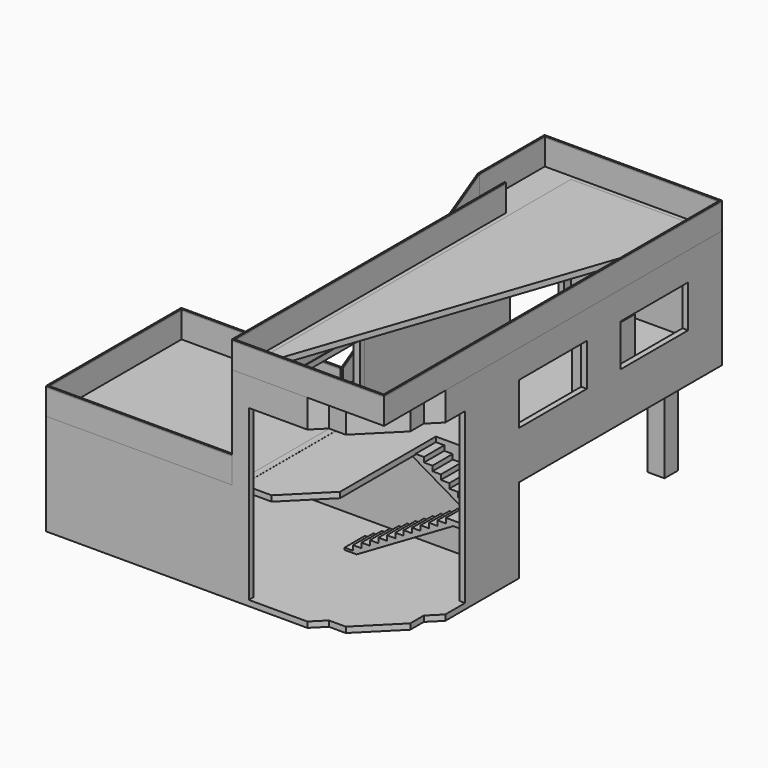
from build123d import *

# Parameters (mm, degrees)
F0_W      = 12192
F0_H      = 6096
F1_DEPTH  = 3657.6
F2_W      = 5486.4
F2_H      = 9144
F2_H_2    = 6096
F3_DEPTH  = 3657.6
F4_W      = 304.8
F4_H      = 101.6
F4_W_2    = 2997.2
F4_H_2    = 203.2
F5_DEPTH  = 914.4
F7_DEPTH  = 914.4
F8_DEPTH  = 50.8
F10_DEPTH = 914.4
F11_DEPTH = 50.8
F13_DEPTH = 50.8
F14_W     = 4876.8
F14_H     = 2438.4
F15_DEPTH = 228.6
F16_T     = -203.2
F17_W     = 3657.6
F17_H     = 6096
F18_DEPTH = 4876.8
F19_W     = 3048
F19_H     = 1524
F20_DEPTH = 203.2
F21_DEPTH = 609.6
F22_DEPTH = 203.2
F24_DEPTH = 203.2
F26_W     = 609.6
F26_H     = 609.6
F27_DEPTH = 3048
F28_W     = 2438.4
F28_H     = 3454.4
F29_DEPTH = 203.2
F30_DEPTH = 50.8
F31_W     = 228.6
F31_H     = 4876.8
F32_DEPTH = 2.54
F34_DEPTH = 7315.201
F36_DEPTH = 812.8
F38_DEPTH = 1828.8
F39_W     = 2090.0571428571
F39_H     = 914.4
F40_DEPTH = 1244.6
F41_W     = 4470.4
F41_H     = 914.4
F42_DEPTH = 2032
F44_DEPTH = 203.2
F46_DEPTH = 203.2
F49_DEPTH = 2438.4


with BuildPart() as f1:
    # F0 (on Top) → F1 (new body)
    with BuildSketch(Plane.XY):
        with Locations((-6096, 3048)):
            Rectangle(F0_W, F0_H)
    extrude(amount=F1_DEPTH)

    # F2 (on face) → F3 (join)
    with BuildSketch(Plane.XY.offset(3657.6)):
        with Locations((-2743.2, 10668)):
            Rectangle(F2_W, F2_H)
        with Locations((-2743.2, 3048)):
            Rectangle(F2_W, F2_H_2)
    extrude(amount=F3_DEPTH)

    # F4 (on face) → F5 (join)
    with BuildSketch(Plane(origin=(-5486.4, 0, 0), x_dir=(0, -1, 0), z_dir=(-1, 0, 0))):
        with Locations((-6248.4, 3784.6)):
            Rectangle(F4_W, F4_H)
        with Locations((-6553.2, 3962.4)):
            Rectangle(F4_W, F4_H)
        with Locations((-6858, 4140.2)):
            Rectangle(F4_W, F4_H)
        with Locations((-7162.8, 4318)):
            Rectangle(F4_W, F4_H)
        with Locations((-7467.6, 4495.8)):
            Rectangle(F4_W, F4_H)
        with Locations((-7772.4, 4673.6)):
            Rectangle(F4_W, F4_H)
        with Locations((-8077.2, 4851.4)):
            Rectangle(F4_W, F4_H)
        with Locations((-8382, 5029.2)):
            Rectangle(F4_W, F4_H)
        with Locations((-8686.8, 5207)):
            Rectangle(F4_W, F4_H)
        with Locations((-8991.6, 5384.8)):
            Rectangle(F4_W, F4_H)
        with Locations((-9296.4, 5562.6)):
            Rectangle(F4_W, F4_H)
        with Locations((-9601.2, 5740.4)):
            Rectangle(F4_W, F4_H)
        with Locations((-9906, 5918.2)):
            Rectangle(F4_W, F4_H)
        with Locations((-10210.8, 6096)):
            Rectangle(F4_W, F4_H)
        with Locations((-10515.6, 6273.8)):
            Rectangle(F4_W, F4_H)
        with Locations((-10820.4, 6451.6)):
            Rectangle(F4_W, F4_H)
        with Locations((-11125.2, 6629.4)):
            Rectangle(F4_W, F4_H)
        with Locations((-11430, 6807.2)):
            Rectangle(F4_W, F4_H)
        with Locations((-11734.8, 6985)):
            Rectangle(F4_W, F4_H)
        with Locations((-12039.6, 7162.8)):
            Rectangle(F4_W, F4_H)
        with Locations((-13741.4, 7213.6)):
            Rectangle(F4_W_2, F4_H_2)
    extrude(amount=F5_DEPTH)

    # F14 (on face) → F15 (cut)
    with BuildSketch(Plane(origin=(-5486.4, 0, 0), x_dir=(0, -1, 0), z_dir=(-1, 0, 0))):
        with Locations((-3048, 4876.8)):
            Rectangle(F14_W, F14_H)
    extrude(amount=-F15_DEPTH, mode=Mode.SUBTRACT)

    # F16: a shell. OpenCascade refuses it in one call, so the cavity is built on its own and cut out:
    # the body offset inwards by the wall thickness, plus a prism from it out through each open face.
    f16_core = offset(f1.part, amount=F16_T, kind=Kind.INTERSECTION, mode=Mode.PRIVATE)
    f16_exits = [f16_core.faces().sort_by_distance(p)[0] for p in [
        (-5054.6, 3048, 4876.8),
    ]]
    add(f16_core, mode=Mode.SUBTRACT)
    extrude(f16_exits, amount=-F16_T, mode=Mode.SUBTRACT)

    # F17 (on face) → F18 (cut)
    with BuildSketch(Plane.YZ):
        with Locations((1828.8, 3251.2)):
            Rectangle(F17_W, F17_H)
    extrude(amount=-F18_DEPTH, mode=Mode.SUBTRACT)

    # F19 (on face) → F20 (cut, through all)
    with BuildSketch(Plane.YZ):
        with Locations((7620, 5537.2)):
            Rectangle(F19_W, F19_H)
        with Locations((12192, 5537.2)):
            Rectangle(F19_W, F19_H)
    extrude(amount=-F20_DEPTH, mode=Mode.SUBTRACT)

    # F21 (add): a face of the model
    f21_faces = [f1.faces().sort_by_distance(p)[0] for p in [
        (-2743.2, 10668, 3657.6),
    ]]
    extrude(f21_faces, amount=F21_DEPTH)

    # F22 (cut): a face of the model
    f22_faces = [f1.faces().sort_by_distance(p)[0] for p in [
        (-2743.2, 10464.8, 3860.8),
    ]]
    extrude(f22_faces, amount=-F22_DEPTH, mode=Mode.SUBTRACT)

    # F23 (on face) → F24 (join)
    with BuildSketch(Plane.XY.offset(3657.6)):
        Polygon((-2844.8, 5892.8), (-5283.2, 5892.8), (-5283.2, 203.2), (-4216.4, 203.2), (-2844.8, 1574.8), align=None)
    extrude(amount=-F24_DEPTH)

    # F28 (on face) → F29 (cut, through all)
    with BuildSketch(Plane.YZ.offset(-5283.2)):
        with Locations((13512.8, 5384.8)):
            Rectangle(F28_W, F28_H)
    extrude(amount=-F29_DEPTH, mode=Mode.SUBTRACT)

    # F31 (on face) → F32 (join)
    with BuildSketch(Plane.XY.offset(3657.6)):
        with Locations((-5372.1, 3048)):
            Rectangle(F31_W, F31_H)
    extrude(amount=F32_DEPTH)

    # F33 (on face) → F34 (cut, through all)
    with BuildSketch(Plane.XY.offset(7315.2)):
        Polygon((0, 0), (0, 2764.8614690566), (-431.0522938113, 2333.8091752453), (-431.0522938113, 1724.2091752453), (-1724.2091752453, 431.0522938113), (-2333.8091752453, 431.0522938113), (-2764.8614690566, 0), align=None)
    extrude(amount=-F34_DEPTH, mode=Mode.SUBTRACT)

    # F35 (on face) → F36 (join, through all)
    with BuildSketch(Plane(origin=(0, 0, 7112), x_dir=(1, 0, 0), z_dir=(0, 0, -1))):
        Polygon((-634.2522938113, -1808.3773711195), (-634.2522938113, -2417.9773711195), (-203.2, -2849.0296649308), (-203.2, -2561.6614690566), (-431.0522938113, -2333.8091752453), (-431.0522938113, -1724.2091752453), (-1724.2091752453, -431.0522938113), (-2333.8091752453, -431.0522938113), (-2561.6614690566, -203.2), (-2849.0296649308, -203.2), (-2417.9773711195, -634.2522938113), (-1808.3773711195, -634.2522938113), align=None)
    extrude(amount=F36_DEPTH)

    # F43 (on face) → F44 (cut, through all)
    with BuildSketch(Plane(origin=(0, 0, 7112), x_dir=(1, 0, 0), z_dir=(0, 0, -1))):
        Polygon((-5283.1906064678, -15036.7906064678), (-215.8906064678, -15036.7906064678), (-215.8906064678, -2836.339058463), (-634.2522938113, -2417.9773711195), (-634.2522938113, -1808.3773711195), (-1808.3773711195, -634.2522938113), (-2417.9773711195, -634.2522938113), (-2836.339058463, -215.8906064678), (-5283.1906064678, -215.8906064678), align=None)
    extrude(amount=-F44_DEPTH, mode=Mode.SUBTRACT)


with BuildPart() as f7:
    # F6 (on face) → F7 (new body)
    with BuildSketch(Plane.XY.offset(3657.6)):
        Polygon((-5486.4, 0), (-5486.4, 50.8001289368), (-12141.1998710632, 50.8001289368), (-12141.1998710632, 6045.1998710632), (-6400.8, 6045.1998710632), (-6400.8, 6096), (-12192, 6096), (-12192, 0), align=None)
    extrude(amount=F7_DEPTH)


with BuildPart() as f8:
    # F8 (new): a face of the model
    f8_faces = [f7.part.faces().sort_by_distance(p)[0] for p in [
        (-5577.0235550837, 25.4000644684, 4572),
    ]]
    extrude(f8_faces, amount=F8_DEPTH)


with BuildPart() as f10:
    # F9 (on face) → F10 (new body)
    with BuildSketch(Plane.XY.offset(7315.2)):
        Polygon((-50.8002166748, 15189.1997833252), (-50.8002166748, 50.8002166748), (-5435.5997833252, 50.8002166748), (-5435.5997833252, 12293.6002166748), (-5486.4, 12293.6002166748), (-5486.4, 12242.8), (-5486.4, 0), (0, 0), (0, 15240), (-6400.8, 15240), (-6400.8, 12242.8), (-6349.9997833252, 12242.8), (-6349.9997833252, 12293.6002166748), (-6349.9997833252, 15189.1997833252), align=None)
    extrude(amount=F10_DEPTH)


with BuildPart() as f11:
    # F11 (new): a face of the model
    f11_faces = [f10.part.faces().sort_by_distance(p)[0] for p in [
        (-6366.5293883005, 13715.9998916626, 8229.6),
    ]]
    extrude(f11_faces, amount=F11_DEPTH)


with BuildPart() as f13:
    # F12 (on face) → F13 (new body)
    with BuildSketch(Plane(origin=(-6400.8, 0, 0), x_dir=(0, -1, 0), z_dir=(-1, 0, 0))):
        Polygon((-11901.3111111111, 7112), (-6096, 3657.6), (-6096, 4572), (-12242.8, 8229.6), (-12242.8, 7315.2), (-12072.0555555556, 7213.6), (-11887.2, 7213.6), (-11887.2, 7112), align=None)
    extrude(amount=-F13_DEPTH)


with BuildPart() as f27:
    # F26 (on face) → F27 (new body, through all)
    with BuildSketch(Plane(origin=(0, 0, 3048), x_dir=(1, 0, 0), z_dir=(0, 0, -1))):
        with Locations((-914.4, -13716)):
            Rectangle(F26_W, F26_H)
    extrude(amount=F27_DEPTH)


with BuildPart() as f27b:
    # F26 (on face) → F27, piece 2 (new body, through all)
    with BuildSketch(Plane(origin=(0, 0, 3048), x_dir=(1, 0, 0), z_dir=(0, 0, -1))):
        with Locations((-4572, -13716)):
            Rectangle(F26_W, F26_H)
    extrude(amount=F27_DEPTH)


with BuildPart() as f30:
    # F30 (new): a face of the model
    f30_faces = [f13.part.faces().sort_by_distance(p)[0] for p in [
        (-6375.4, 9169.4, 6400.8),
    ]]
    extrude(f30_faces, amount=F30_DEPTH)


with BuildPart() as f38:
    # F37 (on face) → F38 (new body)
    with BuildSketch(Plane.XZ.offset(-5892.8)):
        Polygon((-2540, 3479.8), (-2844.8, 3479.8), (-2844.8, 3454.4), (-3106.0571428571, 3454.4), (-1016, 2235.2), (-1320.8, 2235.2), (-1320.8, 2057.4), (-1625.6, 2057.4), (-1625.6, 1879.6), (-1930.4, 1879.6), (-1930.4, 1701.8), (-2235.2, 1701.8), (-2235.2, 1524), (-2540, 1524), (-2540, 1346.2), (-2844.8, 1346.2), (-2844.8, 1168.4), (-3149.6, 1168.4), (-3149.6, 990.6), (-3454.4, 990.6), (-3454.4, 812.8), (-3759.2, 812.8), (-3759.2, 635), (-4064, 635), (-4064, 457.2), (-4368.8, 457.2), (-4368.8, 279.4), (-4673.6, 279.4), (-4673.6, 203.2), (-4238.1714285714, 203.2), (-754.7428571429, 2235.2), (-203.2, 2235.2), (-203.2, 2413), (-1016, 2413), (-1016, 2590.8), (-1320.8, 2590.8), (-1320.8, 2768.6), (-1625.6, 2768.6), (-1625.6, 2946.4), (-1930.4, 2946.4), (-1930.4, 3124.2), (-2235.2, 3124.2), (-2235.2, 3302), (-2540, 3302), align=None)
    extrude(amount=F38_DEPTH)

    # F39 (on face) → F40 (cut, through all)
    with BuildSketch(Plane.XY.offset(3479.8)):
        with Locations((-2061.0285714286, 4521.2)):
            Rectangle(F39_W, F39_H)
    extrude(amount=-F40_DEPTH, mode=Mode.SUBTRACT)

    # F41 (on face) → F42 (cut, through all)
    with BuildSketch(Plane(origin=(0, 0, 2235.2), x_dir=(1, 0, 0), z_dir=(0, 0, -1))):
        with Locations((-2438.4, -5435.6)):
            Rectangle(F41_W, F41_H)
    extrude(amount=F42_DEPTH, mode=Mode.SUBTRACT)


with BuildPart() as f46:
    # F45 (on face) → F46 (new body)
    with BuildSketch(Plane.XY.offset(7315.2)):
        Polygon((-5283.1906064678, 215.8906064678), (-215.8906064678, 15036.7906064678), (-5283.1906064678, 15036.7906064678), align=None)
    extrude(amount=-F46_DEPTH)


with BuildPart() as f49:
    # F48 (on face) → F49 (new body)
    with BuildSketch(Plane.XY.offset(3657.6)):
        Polygon((-1270, 10058.4), (-203.2, 10058.4), (-203.2, 11582.4), (-695.2636082516, 11582.4), (-1270, 11007.6636082516), align=None)
    extrude(amount=F49_DEPTH)


solid = Compound([f1.part, f7.part, f8.part, f10.part, f11.part, f13.part, f27.part, f27b.part, f30.part, f38.part, f46.part, f49.part])
